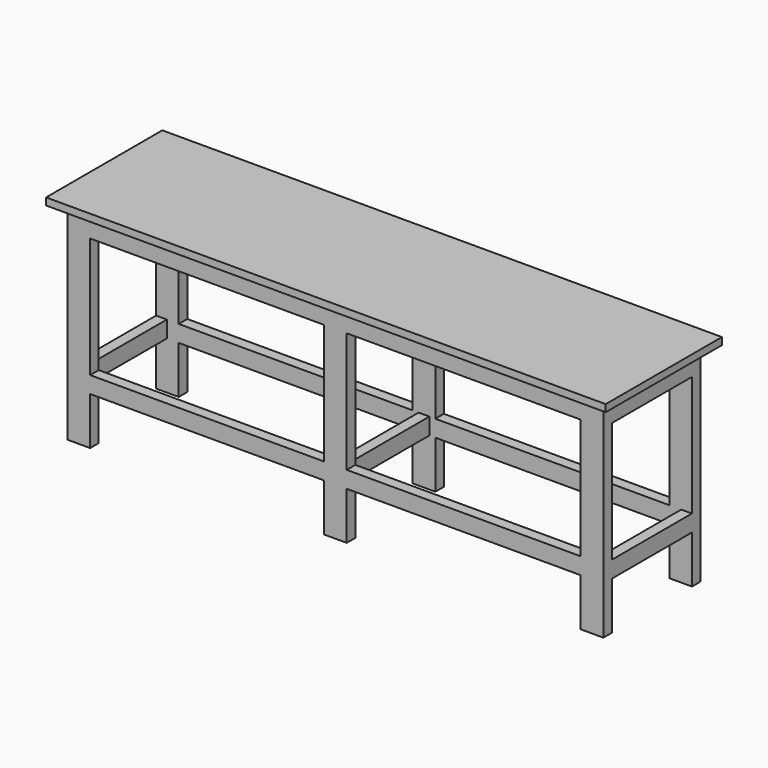
from build123d import *

# Parameters (mm, degrees)
F1_W     = 2350
F1_H     = 610
F2_DEPTH = 30
F3_W     = 45
F3_H     = 420
F3_W_2   = 982.5
F3_H_2   = 45
F4_DEPTH = 95
F5_DEPTH = 870
F7_W     = 982.5
F7_H     = 45
F7_W_2   = 45
F7_H_2   = 420
F8_DEPTH = 70


# Not quite as in the source:
# - a feature names something its author has since deleted; it is built from what else it names


with BuildPart() as f2:
    # F1 (on offset) → F2 (new body)
    with BuildSketch(Plane.XY.offset(900)):
        Rectangle(F1_W, F1_H)
    extrude(amount=-F2_DEPTH)

    # F3 (on face) → F4 (join)
    with BuildSketch(Plane(origin=(0, 0, 870), x_dir=(1, 0, 0), z_dir=(0, 0, -1))):
        with Locations((-1102.5, 0)):
            Rectangle(F3_W, F3_H)
        with Locations((1102.5, 0)):
            Rectangle(F3_W, F3_H)
        with Locations((-538.75, 232.5)):
            Rectangle(F3_W_2, F3_H_2)
        with Locations((-538.75, -232.5)):
            Rectangle(F3_W_2, F3_H_2)
        Polygon((22.5, 210), (-22.5, 210), (-22.5, -210), (22.5, -210), (22.5, -47.5), (22.5, 47.5), align=None)
        with Locations((538.75, 232.5)):
            Rectangle(F3_W_2, F3_H_2)
        with Locations((538.75, -232.5)):
            Rectangle(F3_W_2, F3_H_2)
    extrude(amount=F4_DEPTH)

    # F3 (on face) → F5 (join)
    with BuildSketch(Plane(origin=(0, 0, 870), x_dir=(1, 0, 0), z_dir=(0, 0, -1))):
        Polygon((-1030, 255), (-1125, 255), (-1125, 210), (-1080, 210), (-1030, 210), align=None)
        Polygon((47.5, 255), (-47.5, 255), (-47.5, 210), (-22.5, 210), (22.5, 210), (47.5, 210), align=None)
        Polygon((-1080, -210), (-1125, -210), (-1125, -255), (-1030, -255), (-1030, -210), align=None)
        Polygon((1125, 255), (1030, 255), (1030, 210), (1080, 210), (1125, 210), align=None)
        Polygon((22.5, -210), (-22.5, -210), (-47.5, -210), (-47.5, -255), (47.5, -255), (47.5, -210), align=None)
        Polygon((1125, -210), (1080, -210), (1030, -210), (1030, -255), (1125, -255), align=None)
    extrude(amount=F5_DEPTH)

    # F7 (on offset) → F8 (join)
    with BuildSketch(Plane.XY.offset(200)):
        with Locations((-538.75, 232.5)):
            Rectangle(F7_W, F7_H)
        Polygon((22.5, 255), (-47.5, 255), (-47.5, 210), (-22.5, 210), (22.5, 210), (47.5, 210), (47.5, 255), align=None)
        Polygon((67.5, 255), (47.5, 255), (47.5, 210), (67.5, 210), (1030, 210), (1030, 255), align=None)
        Polygon((22.5, 210), (-22.5, 210), (-22.5, -210), (22.5, -210), (22.5, -47.5), (22.5, 47.5), align=None)
        Polygon((22.5, -210), (-22.5, -210), (-47.5, -210), (-47.5, -255), (22.5, -255), (47.5, -255), (47.5, -210), align=None)
        with Locations((-538.75, -232.5)):
            Rectangle(F7_W, F7_H)
        Polygon((67.5, -210), (47.5, -210), (47.5, -255), (1030, -255), (1030, -210), align=None)
        with Locations((-1102.5, 0)):
            Rectangle(F7_W_2, F7_H_2)
        with Locations((1102.5, 0)):
            Rectangle(F7_W_2, F7_H_2)
    extrude(amount=F8_DEPTH)


solid = f2.part
